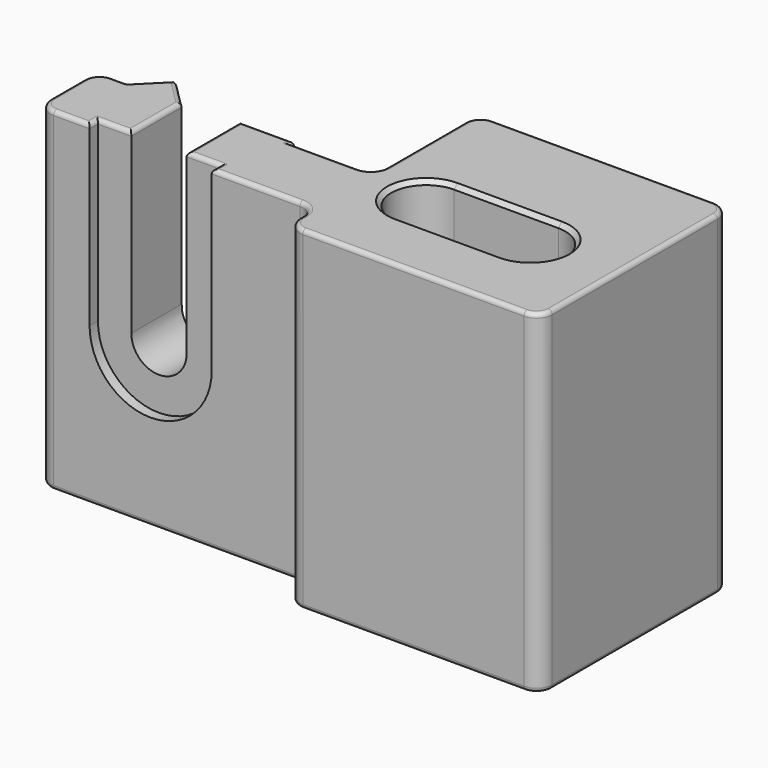
from build123d import *

# Parameters (mm, degrees)
F1_DEPTH      = 32
F2_R          = 0.4
F3_R          = 1.5
F5_DEPTH      = 19.401
F6_DEPTH      = 1
F7_T1_DEPTH   = 1.2843145751
F7_T3_DEPTH   = 4.0870057685
F7_T5_DEPTH   = 4.0870057685
F7_T7_DEPTH   = 8.0359281116
F7_T9_DEPTH   = 4.2
F7_T11_DEPTH  = 2
F7_T13_DEPTH  = 4.45
F7_T15_DEPTH  = 4
F7_T17_DEPTH  = 6.5
F7_T19_DEPTH  = 1.4
F7_T21_DEPTH  = 9.4
F7_T23_DEPTH  = 7.15
F7_T25_DEPTH  = 21.2
F7_T27_DEPTH  = 5.1343145751
F7_T29_DEPTH  = 19.8
F7_T31_DEPTH  = 0.4
F7_T33_DEPTH  = 23.6
F7_T35_DEPTH  = 8.4
F7_T37_DEPTH  = 9.45
F7_T39_DEPTH  = 4.2
F7_T42_ANGLE  = 90
F7_T44_ANGLE  = 90
F7_T46_ANGLE  = 90
F7_T48_ANGLE  = 90
F7_T50_ANGLE  = 90
F7_T52_ANGLE  = 45
F7_T54_ANGLE  = 90
F7_T56_ANGLE  = 90
F7_T58_ANGLE  = 45
F7_T60_ANGLE  = 90
F7_T62_ANGLE  = 90
F7_T64_ANGLE  = 90
F7_T66_ANGLE  = 90
F7_T68_ANGLE  = 90
F7_T70_ANGLE  = 90
F7_T72_ANGLE  = 163.7726416214
F7_T74_ANGLE  = 90
F7_T76_ANGLE  = 90
F7_T78_ANGLE  = 45
F7_T80_ANGLE  = 90
F7_T85_DEPTH  = 5.2
F7_T89_DEPTH  = 3
F7_T96_DEPTH  = 7.5
F7_T100_DEPTH = 2.4
F7_T107_DEPTH = 2.4
F7_T111_DEPTH = 6.1343145751
F7_T118_DEPTH = 7.5
F7_T122_DEPTH = 2.4
F7_T129_DEPTH = 3
F7_T133_DEPTH = 5.2
F10_SIZE      = 0.4
F11_SIZE      = 0.4


# Not quite as in the source:
# - a fillet or chamfer that OpenCascade refuses, or shapes differently, is made with other operations: its cross-section is extruded or revolved along the edge and cut away or added
# - two fillets or chamfers of one size are made in one step


with BuildPart() as f1:
    # F0 (on Top) → F1 (new body)
    with BuildSketch(Plane.XY):
        Polygon((-7.85, 0), (-10.8, 0), (-10.8, -7), (15.8, -7), (15.8, -10.4), (40, -10.4), (40, 12.4), (15.8, 12.4), (15.8, 0), (7.8, 0), (7.8, 0.4), (2.65, 0.4), (2.65, 0), (-2.65, 0), (-4.95, 2.3), (-5.55, 2.3), align=None)
        with BuildLine():
            ThreePointArc((21.6, -4.35), (18.25, -1), (21.6, 2.35))
            Line((21.6, 2.35), (31.6, 2.35))
            ThreePointArc((31.6, 2.35), (34.95, -1), (31.6, -4.35))
            Line((31.6, -4.35), (21.6, -4.35))
        make_face(mode=Mode.SUBTRACT)
    extrude(amount=F1_DEPTH)

    # F2
    f2_edges = [f1.edges().sort_by_distance(p)[0] for p in [
        (-7.85, 0, 16),
        (-2.65, 0, 16),
    ]]
    fillet(f2_edges, radius=F2_R)

    # F3
    f3_edges = [f1.edges().sort_by_distance(p)[0] for p in [
        (-10.8, 0, 16),
        (-10.8, -7, 16),
        (15.8, 12.4, 16),
        (40, 12.4, 16),
        (15.8, -10.4, 16),
        (40, -10.4, 16),
        (15.8, -7, 16),
        (15.8, 0, 16),
    ]]
    fillet(f3_edges, radius=F3_R)

    # F4 (on face) → F5 (cut, through all)
    with BuildSketch(Plane.XZ.offset(7)):
        with BuildLine():
            Line((2.65, 15), (2.65, 32))
            Line((2.65, 32), (-2.65, 32))
            Line((-2.65, 32), (-2.65, 15))
            ThreePointArc((-2.65, 15), (0, 12.35), (2.65, 15))
        make_face()
    extrude(amount=-F5_DEPTH, mode=Mode.SUBTRACT)

    # F4 (on face) → F6 (cut)
    with BuildSketch(Plane.XZ.offset(7)):
        with BuildLine():
            Line((5.85, 32), (2.65, 32))
            Line((2.65, 32), (2.65, 15))
            ThreePointArc((2.65, 15), (0, 12.35), (-2.65, 15))
            Line((-2.65, 15), (-2.65, 32))
            Line((-2.65, 32), (-5.85, 32))
            Line((-5.85, 32), (-5.85, 15))
            ThreePointArc((-5.85, 15), (0, 9.15), (5.85, 15))
            Line((5.85, 15), (5.85, 32))
        make_face()
    extrude(amount=-F6_DEPTH, mode=Mode.SUBTRACT)

    # F7: fillet of radius 0.4 on 55 edges, made by hand

    # F7_s2 → F7_t1 (cut)
    with BuildSketch(Plane.YZ.offset(-9.3)):
        with BuildLine():
            ThreePointArc((0, 31.6), (-0.1171572875, 31.8828427125), (-0.4, 32))
            Line((-0.4, 32), (0, 32))
            Line((0, 32), (0, 31.6))
        make_face()
        with BuildLine():
            ThreePointArc((-0.4, 0), (-0.1171572875, 0.1171572875), (0, 0.4))
            Line((0, 0.4), (0, 0))
            Line((0, 0), (-0.4, 0))
        make_face()
    extrude(amount=F7_T1_DEPTH, mode=Mode.SUBTRACT)

    # F7_s4 → F7_t3 (cut)
    with BuildSketch(Plane(origin=(-0.9178932188, -0.9178932188, 0), x_dir=(0, 0, 1), z_dir=(-0.7071067812, -0.7071067812, 0))):
        with BuildLine():
            ThreePointArc((31.6, 5.5507882323), (31.8828427125, 5.4336309448), (32, 5.1507882323))
            Line((32, 5.1507882323), (32, 5.5507882323))
            Line((32, 5.5507882323), (31.6, 5.5507882323))
        make_face()
        with BuildLine():
            ThreePointArc((0, 5.1507882323), (0.1171572875, 5.4336309448), (0.4, 5.5507882323))
            Line((0.4, 5.5507882323), (0, 5.5507882323))
            Line((0, 5.5507882323), (0, 5.1507882323))
        make_face()
    extrude(amount=F7_T3_DEPTH, mode=Mode.SUBTRACT)

    # F7_s6 → F7_t5 (cut)
    with BuildSketch(Plane(origin=(-1.4421572875, 1.4421572875, 0), x_dir=(0, 0, 1), z_dir=(-0.7071067812, 0.7071067812, 0))):
        with BuildLine():
            ThreePointArc((31.6, -1.8738329701), (31.8828427125, -1.9909902577), (32, -2.2738329701))
            Line((32, -2.2738329701), (32, -1.8738329701))
            Line((32, -1.8738329701), (31.6, -1.8738329701))
        make_face()
        with BuildLine():
            ThreePointArc((0, -2.2738329701), (0.1171572875, -1.9909902577), (0.4, -1.8738329701))
            Line((0.4, -1.8738329701), (0, -1.8738329701))
            Line((0, -1.8738329701), (0, -2.2738329701))
        make_face()
    extrude(amount=F7_T5_DEPTH, mode=Mode.SUBTRACT)

    # F7_s8 → F7_t7 (cut)
    with BuildSketch(Plane.XZ.offset(-1.0359281116)):
        with BuildLine():
            ThreePointArc((-2.65, 31.6), (-2.7671572875, 31.8828427125), (-3.05, 32))
            Line((-3.05, 32), (-2.65, 32))
            Line((-2.65, 32), (-2.65, 31.6))
        make_face()
    extrude(amount=F7_T7_DEPTH, mode=Mode.SUBTRACT)

    # F7_s10 → F7_t9 (cut)
    with BuildSketch(Plane.YZ.offset(-5.85)):
        with BuildLine():
            ThreePointArc((-6, 31.6), (-5.8828427125, 31.8828427125), (-5.6, 32))
            Line((-5.6, 32), (-6, 32))
            Line((-6, 32), (-6, 31.6))
        make_face()
    extrude(amount=F7_T9_DEPTH, mode=Mode.SUBTRACT)

    # F7_s12 → F7_t11 (cut)
    with BuildSketch(Plane.XZ.offset(6)):
        with BuildLine():
            ThreePointArc((-6.25, 32), (-5.9671572875, 31.8828427125), (-5.85, 31.6))
            Line((-5.85, 31.6), (-5.85, 32))
            Line((-5.85, 32), (-6.25, 32))
        make_face()
        with BuildLine():
            ThreePointArc((6.25, 32), (5.9671572875, 31.8828427125), (5.85, 31.6))
            Line((5.85, 31.6), (5.85, 32))
            Line((5.85, 32), (6.25, 32))
        make_face()
    extrude(amount=F7_T11_DEPTH, mode=Mode.SUBTRACT)

    # F7_s14 → F7_t13 (cut)
    with BuildSketch(Plane.YZ.offset(-9.3)):
        with BuildLine():
            ThreePointArc((-7, 31.6), (-6.8828427125, 31.8828427125), (-6.6, 32))
            Line((-6.6, 32), (-7, 32))
            Line((-7, 32), (-7, 31.6))
        make_face()
    extrude(amount=F7_T13_DEPTH, mode=Mode.SUBTRACT)

    # F7_s16 → F7_t15 (cut)
    with BuildSketch(Plane.XZ.offset(1.5)):
        with BuildLine():
            ThreePointArc((-10.8, 31.6), (-10.6828427125, 31.8828427125), (-10.4, 32))
            Line((-10.4, 32), (-10.8, 32))
            Line((-10.8, 32), (-10.8, 31.6))
        make_face()
        with BuildLine():
            ThreePointArc((-10.4, 0), (-10.6828427125, 0.1171572875), (-10.8, 0.4))
            Line((-10.8, 0.4), (-10.8, 0))
            Line((-10.8, 0), (-10.4, 0))
        make_face()
    extrude(amount=F7_T15_DEPTH, mode=Mode.SUBTRACT)

    # F7_s18 → F7_t17 (cut)
    with BuildSketch(Plane.YZ.offset(7.8)):
        with BuildLine():
            ThreePointArc((-0.4, 0), (-0.1171572875, 0.1171572875), (0, 0.4))
            Line((0, 0.4), (0, 0))
            Line((0, 0), (-0.4, 0))
        make_face()
        with BuildLine():
            ThreePointArc((0, 31.6), (-0.1171572875, 31.8828427125), (-0.4, 32))
            Line((-0.4, 32), (0, 32))
            Line((0, 32), (0, 31.6))
        make_face()
    extrude(amount=F7_T17_DEPTH, mode=Mode.SUBTRACT)

    # F7_s20 → F7_t19 (cut)
    with BuildSketch(Plane.XZ.offset(-1.4)):
        with BuildLine():
            ThreePointArc((7.4, 0), (7.6828427125, 0.1171572875), (7.8, 0.4))
            Line((7.8, 0.4), (7.8, 0))
            Line((7.8, 0), (7.4, 0))
        make_face()
        with BuildLine():
            ThreePointArc((3.05, 0), (2.7671572875, 0.1171572875), (2.65, 0.4))
            Line((2.65, 0.4), (2.65, 0))
            Line((2.65, 0), (3.05, 0))
        make_face()
        with BuildLine():
            ThreePointArc((7.8, 31.6), (7.6828427125, 31.8828427125), (7.4, 32))
            Line((7.4, 32), (7.8, 32))
            Line((7.8, 32), (7.8, 31.6))
        make_face()
    extrude(amount=F7_T19_DEPTH, mode=Mode.SUBTRACT)

    # F7_s22 → F7_t21 (cut)
    with BuildSketch(Plane.XZ.offset(-10.9)):
        with BuildLine():
            ThreePointArc((16.2, 0), (15.9171572875, 0.1171572875), (15.8, 0.4))
            Line((15.8, 0.4), (15.8, 0))
            Line((15.8, 0), (16.2, 0))
        make_face()
        with BuildLine():
            ThreePointArc((15.8, 31.6), (15.9171572875, 31.8828427125), (16.2, 32))
            Line((16.2, 32), (15.8, 32))
            Line((15.8, 32), (15.8, 31.6))
        make_face()
    extrude(amount=F7_T21_DEPTH, mode=Mode.SUBTRACT)

    # F7_s24 → F7_t23 (cut)
    with BuildSketch(Plane.YZ.offset(1.65)):
        with BuildLine():
            ThreePointArc((0, 0), (0.2828427125, 0.1171572875), (0.4, 0.4))
            Line((0.4, 0.4), (0.4, 0))
            Line((0.4, 0), (0, 0))
        make_face()
        with BuildLine():
            ThreePointArc((0.4, 31.6), (0.2828427125, 31.8828427125), (0, 32))
            Line((0, 32), (0.4, 32))
            Line((0.4, 32), (0.4, 31.6))
        make_face()
    extrude(amount=F7_T23_DEPTH, mode=Mode.SUBTRACT)

    # F7_s26 → F7_t25 (cut)
    with BuildSketch(Plane.YZ.offset(17.3)):
        with BuildLine():
            ThreePointArc((12, 0), (12.2828427125, 0.1171572875), (12.4, 0.4))
            Line((12.4, 0.4), (12.4, 0))
            Line((12.4, 0), (12, 0))
        make_face()
        with BuildLine():
            ThreePointArc((-10, 0), (-10.2828427125, 0.1171572875), (-10.4, 0.4))
            Line((-10.4, 0.4), (-10.4, 0))
            Line((-10.4, 0), (-10, 0))
        make_face()
        with BuildLine():
            ThreePointArc((12.4, 31.6), (12.2828427125, 31.8828427125), (12, 32))
            Line((12, 32), (12.4, 32))
            Line((12.4, 32), (12.4, 31.6))
        make_face()
        with BuildLine():
            ThreePointArc((-10.4, 31.6), (-10.2828427125, 31.8828427125), (-10, 32))
            Line((-10, 32), (-10.4, 32))
            Line((-10.4, 32), (-10.4, 31.6))
        make_face()
    extrude(amount=F7_T25_DEPTH, mode=Mode.SUBTRACT)

    # F7_s28 → F7_t27 (cut)
    with BuildSketch(Plane.YZ.offset(-2.4843145751)):
        with BuildLine():
            ThreePointArc((-0.4, 0), (-0.1171572875, 0.1171572875), (0, 0.4))
            Line((0, 0.4), (0, 0))
            Line((0, 0), (-0.4, 0))
        make_face()
    extrude(amount=F7_T27_DEPTH, mode=Mode.SUBTRACT)

    # F7_s30 → F7_t29 (cut)
    with BuildSketch(Plane.XZ.offset(-10.9)):
        with BuildLine():
            ThreePointArc((39.6, 0), (39.8828427125, 0.1171572875), (40, 0.4))
            Line((40, 0.4), (40, 0))
            Line((40, 0), (39.6, 0))
        make_face()
        with BuildLine():
            ThreePointArc((40, 31.6), (39.8828427125, 31.8828427125), (39.6, 32))
            Line((39.6, 32), (40, 32))
            Line((40, 32), (40, 31.6))
        make_face()
    extrude(amount=F7_T29_DEPTH, mode=Mode.SUBTRACT)

    # F7_s32 → F7_t31 (cut)
    with BuildSketch(Plane.XZ.offset(8.5)):
        with BuildLine():
            ThreePointArc((16.2, 0), (15.9171572875, 0.1171572875), (15.8, 0.4))
            Line((15.8, 0.4), (15.8, 0))
            Line((15.8, 0), (16.2, 0))
        make_face()
        with BuildLine():
            ThreePointArc((15.8, 31.6), (15.9171572875, 31.8828427125), (16.2, 32))
            Line((16.2, 32), (15.8, 32))
            Line((15.8, 32), (15.8, 31.6))
        make_face()
    extrude(amount=F7_T31_DEPTH, mode=Mode.SUBTRACT)

    # F7_s34 → F7_t33 (cut)
    with BuildSketch(Plane.YZ.offset(-9.3)):
        with BuildLine():
            ThreePointArc((-6.6, 0), (-6.8828427125, 0.1171572875), (-7, 0.4))
            Line((-7, 0.4), (-7, 0))
            Line((-7, 0), (-6.6, 0))
        make_face()
    extrude(amount=F7_T33_DEPTH, mode=Mode.SUBTRACT)

    # F7_s36 → F7_t35 (cut)
    with BuildSketch(Plane.XZ.offset(-1.4)):
        with BuildLine():
            ThreePointArc((2.65, 31.6), (2.7671572875, 31.8828427125), (3.05, 32))
            Line((3.05, 32), (2.65, 32))
            Line((2.65, 32), (2.65, 31.6))
        make_face()
    extrude(amount=F7_T35_DEPTH, mode=Mode.SUBTRACT)

    # F7_s38 → F7_t37 (cut)
    with BuildSketch(Plane.YZ.offset(4.85)):
        with BuildLine():
            ThreePointArc((-7, 31.6), (-6.8828427125, 31.8828427125), (-6.6, 32))
            Line((-6.6, 32), (-7, 32))
            Line((-7, 32), (-7, 31.6))
        make_face()
    extrude(amount=F7_T37_DEPTH, mode=Mode.SUBTRACT)

    # F7_s40 → F7_t39 (cut)
    with BuildSketch(Plane.YZ.offset(1.65)):
        with BuildLine():
            ThreePointArc((-5.6, 32), (-5.8828427125, 31.8828427125), (-6, 31.6))
            Line((-6, 31.6), (-6, 32))
            Line((-6, 32), (-5.6, 32))
        make_face()
    extrude(amount=F7_T39_DEPTH, mode=Mode.SUBTRACT)

    # F7_s41 → F7_t42 (revolve, cut)
    with BuildSketch(Plane.YZ.offset(-9.3)):
        with BuildLine():
            ThreePointArc((0, 31.6), (-0.1171572875, 31.8828427125), (-0.4, 32))
            Line((-0.4, 32), (0, 32))
            Line((0, 32), (0, 31.6))
        make_face()
    revolve(axis=Axis((-9.3, -1.5, 32), (0, 0, 1)), revolution_arc=F7_T42_ANGLE, mode=Mode.SUBTRACT)

    # F7_s43 → F7_t44 (revolve, cut)
    with BuildSketch(Plane.XZ.offset(5.5)):
        with BuildLine():
            ThreePointArc((-10.8, 31.6), (-10.6828427125, 31.8828427125), (-10.4, 32))
            Line((-10.4, 32), (-10.8, 32))
            Line((-10.8, 32), (-10.8, 31.6))
        make_face()
    revolve(axis=Axis((-9.3, -5.5, 32), (0, 0, 1)), revolution_arc=F7_T44_ANGLE, mode=Mode.SUBTRACT)

    # F7_s45 → F7_t46 (revolve, cut)
    with BuildSketch(Plane.YZ.offset(14.3)):
        with BuildLine():
            ThreePointArc((-0.4, 0), (-0.1171572875, 0.1171572875), (0, 0.4))
            Line((0, 0.4), (0, 0))
            Line((0, 0), (-0.4, 0))
        make_face()
    revolve(axis=Axis((14.3, 1.5, 0), (0, 0, 1)), revolution_arc=F7_T46_ANGLE, mode=Mode.SUBTRACT)

    # F7_s47 → F7_t48 (revolve, cut)
    with BuildSketch(Plane.XZ.offset(-10.9)):
        with BuildLine():
            ThreePointArc((16.2, 0), (15.9171572875, 0.1171572875), (15.8, 0.4))
            Line((15.8, 0.4), (15.8, 0))
            Line((15.8, 0), (16.2, 0))
        make_face()
    revolve(axis=Axis((17.3, 10.9, 0), (0, 0, -1)), revolution_arc=F7_T48_ANGLE, mode=Mode.SUBTRACT)

    # F7_s49 → F7_t50 (revolve, cut)
    with BuildSketch(Plane.YZ.offset(38.5)):
        with BuildLine():
            ThreePointArc((12, 0), (12.2828427125, 0.1171572875), (12.4, 0.4))
            Line((12.4, 0.4), (12.4, 0))
            Line((12.4, 0), (12, 0))
        make_face()
    revolve(axis=Axis((38.5, 10.9, 0), (0, 0, -1)), revolution_arc=F7_T50_ANGLE, mode=Mode.SUBTRACT)

    # F7_s51 → F7_t52 (revolve, cut)
    with BuildSketch(Plane.YZ.offset(-2.4843145751)):
        with BuildLine():
            ThreePointArc((-0.4, 0), (-0.1171572875, 0.1171572875), (0, 0.4))
            Line((0, 0.4), (0, 0))
            Line((0, 0), (-0.4, 0))
        make_face()
    revolve(axis=Axis((-2.4843145751, 0.4, 0), (0, 0, -1)), revolution_arc=F7_T52_ANGLE, mode=Mode.SUBTRACT)

    # F7_s53 → F7_t54 (revolve, cut)
    with BuildSketch(Plane.XZ.offset(8.9)):
        with BuildLine():
            ThreePointArc((39.6, 0), (39.8828427125, 0.1171572875), (40, 0.4))
            Line((40, 0.4), (40, 0))
            Line((40, 0), (39.6, 0))
        make_face()
    revolve(axis=Axis((38.5, -8.9, 0), (0, 0, -1)), revolution_arc=F7_T54_ANGLE, mode=Mode.SUBTRACT)

    # F7_s55 → F7_t56 (revolve, cut)
    with BuildSketch(Plane.YZ.offset(17.3)):
        with BuildLine():
            ThreePointArc((-10, 0), (-10.2828427125, 0.1171572875), (-10.4, 0.4))
            Line((-10.4, 0.4), (-10.4, 0))
            Line((-10.4, 0), (-10, 0))
        make_face()
    revolve(axis=Axis((17.3, -8.9, 0), (0, 0, -1)), revolution_arc=F7_T56_ANGLE, mode=Mode.SUBTRACT)

    # F7_s57 → F7_t58 (revolve, cut)
    with BuildSketch(Plane(origin=(-3.8078427125, -3.8078427125, 0), x_dir=(0, 0, 1), z_dir=(0.7071067812, 0.7071067812, 0))):
        with BuildLine():
            ThreePointArc((0, -5.1507882323), (0.1171572875, -5.4336309448), (0.4, -5.5507882323))
            Line((0.4, -5.5507882323), (0, -5.5507882323))
            Line((0, -5.5507882323), (0, -5.1507882323))
        make_face()
    revolve(axis=Axis((-8.0156854249, 0.4, 0), (0, 0, -1)), revolution_arc=F7_T58_ANGLE, mode=Mode.SUBTRACT)

    # F7_s59 → F7_t60 (revolve, cut)
    with BuildSketch(Plane.YZ.offset(14.3)):
        with BuildLine():
            ThreePointArc((-6.6, 0), (-6.8828427125, 0.1171572875), (-7, 0.4))
            Line((-7, 0.4), (-7, 0))
            Line((-7, 0), (-6.6, 0))
        make_face()
    revolve(axis=Axis((14.3, -8.5, 0), (0, 0, -1)), revolution_arc=F7_T60_ANGLE, mode=Mode.SUBTRACT)

    # F7_s61 → F7_t62 (revolve, cut)
    with BuildSketch(Plane.YZ.offset(-9.3)):
        with BuildLine():
            ThreePointArc((-0.4, 0), (-0.1171572875, 0.1171572875), (0, 0.4))
            Line((0, 0.4), (0, 0))
            Line((0, 0), (-0.4, 0))
        make_face()
    revolve(axis=Axis((-9.3, -1.5, 0), (0, 0, 1)), revolution_arc=F7_T62_ANGLE, mode=Mode.SUBTRACT)

    # F7_s63 → F7_t64 (revolve, cut)
    with BuildSketch(Plane.XZ.offset(5.5)):
        with BuildLine():
            ThreePointArc((-10.4, 0), (-10.6828427125, 0.1171572875), (-10.8, 0.4))
            Line((-10.8, 0.4), (-10.8, 0))
            Line((-10.8, 0), (-10.4, 0))
        make_face()
    revolve(axis=Axis((-9.3, -5.5, 0), (0, 0, 1)), revolution_arc=F7_T64_ANGLE, mode=Mode.SUBTRACT)

    # F7_s65 → F7_t66 (revolve, cut)
    with BuildSketch(Plane.YZ.offset(14.3)):
        with BuildLine():
            ThreePointArc((0, 31.6), (-0.1171572875, 31.8828427125), (-0.4, 32))
            Line((-0.4, 32), (0, 32))
            Line((0, 32), (0, 31.6))
        make_face()
    revolve(axis=Axis((14.3, 1.5, 32), (0, 0, 1)), revolution_arc=F7_T66_ANGLE, mode=Mode.SUBTRACT)

    # F7_s67 → F7_t68 (revolve, cut)
    with BuildSketch(Plane.XZ.offset(-10.9)):
        with BuildLine():
            ThreePointArc((15.8, 31.6), (15.9171572875, 31.8828427125), (16.2, 32))
            Line((16.2, 32), (15.8, 32))
            Line((15.8, 32), (15.8, 31.6))
        make_face()
    revolve(axis=Axis((17.3, 10.9, 32), (0, 0, -1)), revolution_arc=F7_T68_ANGLE, mode=Mode.SUBTRACT)

    # F7_s69 → F7_t70 (revolve, cut)
    with BuildSketch(Plane.YZ.offset(38.5)):
        with BuildLine():
            ThreePointArc((12.4, 31.6), (12.2828427125, 31.8828427125), (12, 32))
            Line((12, 32), (12.4, 32))
            Line((12.4, 32), (12.4, 31.6))
        make_face()
    revolve(axis=Axis((38.5, 10.9, 32), (0, 0, -1)), revolution_arc=F7_T70_ANGLE, mode=Mode.SUBTRACT)

    # F7_s71 → F7_t72 (revolve, cut)
    with BuildSketch(Plane(origin=(-0.7443380199, 1.3554785605, 0), x_dir=(0, 0, 1), z_dir=(-0.4813351882, 0.8765366145, 0))):
        with BuildLine():
            ThreePointArc((31.6, -1.5850586117), (31.8828427125, -1.4679013242), (32, -1.1850586117))
            Line((32, -1.1850586117), (32, -1.5850586117))
            Line((32, -1.5850586117), (31.6, -1.5850586117))
        make_face()
    revolve(axis=Axis((-2.4843145751, 0.4, 32), (0, 0, -1)), revolution_arc=F7_T72_ANGLE, mode=Mode.SUBTRACT)

    # F7_s73 → F7_t74 (revolve, cut)
    with BuildSketch(Plane.XZ.offset(8.9)):
        with BuildLine():
            ThreePointArc((40, 31.6), (39.8828427125, 31.8828427125), (39.6, 32))
            Line((39.6, 32), (40, 32))
            Line((40, 32), (40, 31.6))
        make_face()
    revolve(axis=Axis((38.5, -8.9, 32), (0, 0, -1)), revolution_arc=F7_T74_ANGLE, mode=Mode.SUBTRACT)

    # F7_s75 → F7_t76 (revolve, cut)
    with BuildSketch(Plane.YZ.offset(17.3)):
        with BuildLine():
            ThreePointArc((-10.4, 31.6), (-10.2828427125, 31.8828427125), (-10, 32))
            Line((-10, 32), (-10.4, 32))
            Line((-10.4, 32), (-10.4, 31.6))
        make_face()
    revolve(axis=Axis((17.3, -8.9, 32), (0, 0, -1)), revolution_arc=F7_T76_ANGLE, mode=Mode.SUBTRACT)

    # F7_s77 → F7_t78 (revolve, cut)
    with BuildSketch(Plane(origin=(-3.8078427125, -3.8078427125, 0), x_dir=(0, 0, 1), z_dir=(0.7071067812, 0.7071067812, 0))):
        with BuildLine():
            ThreePointArc((31.6, -5.5507882323), (31.8828427125, -5.4336309448), (32, -5.1507882323))
            Line((32, -5.1507882323), (32, -5.5507882323))
            Line((32, -5.5507882323), (31.6, -5.5507882323))
        make_face()
    revolve(axis=Axis((-8.0156854249, 0.4, 32), (0, 0, -1)), revolution_arc=F7_T78_ANGLE, mode=Mode.SUBTRACT)

    # F7_s79 → F7_t80 (revolve, cut)
    with BuildSketch(Plane.YZ.offset(14.3)):
        with BuildLine():
            ThreePointArc((-7, 31.6), (-6.8828427125, 31.8828427125), (-6.6, 32))
            Line((-6.6, 32), (-7, 32))
            Line((-7, 32), (-7, 31.6))
        make_face()
    revolve(axis=Axis((14.3, -8.5, 32), (0, 0, -1)), revolution_arc=F7_T80_ANGLE, mode=Mode.SUBTRACT)


with BuildPart() as f7_tool83:
    # F7_s84 → F7_t85 (new body)
    with BuildSketch(Plane.YZ.offset(-1.65)):
        with BuildLine():
            ThreePointArc((-6, 31.6), (-5.8828427125, 31.8828427125), (-5.6, 32))
            Line((-5.6, 32), (-6, 32))
            Line((-6, 32), (-6, 31.6))
        make_face()
    extrude(amount=-F7_T85_DEPTH)

    split(bisect_by=Plane.YZ.offset(-5.85), keep=Keep.BOTTOM)


with BuildPart() as f7_tool87:
    # F7_s88 → F7_t89 (new body)
    with BuildSketch(Plane.XZ.offset(8)):
        with BuildLine():
            ThreePointArc((-6.25, 32), (-5.9671572875, 31.8828427125), (-5.85, 31.6))
            Line((-5.85, 31.6), (-5.85, 32))
            Line((-5.85, 32), (-6.25, 32))
        make_face()
    extrude(amount=-F7_T89_DEPTH)

    split(bisect_by=Plane.XZ.offset(6), keep=Keep.BOTTOM)


with BuildPart() as f7_tool83_1:
    add(f7_tool83.part)

    # F7_t91: intersect F7_tool87
    add(f7_tool87.part, mode=Mode.INTERSECT)


with BuildPart() as f1_1:
    add(f1.part)

    # F7_t81: cut F7_tool83
    add(f7_tool83_1.part, mode=Mode.SUBTRACT)


with BuildPart() as f7_tool94:
    # F7_s95 → F7_t96 (new body)
    with BuildSketch(Plane.YZ.offset(14.3)):
        with BuildLine():
            ThreePointArc((-0.4, 0), (-0.1171572875, 0.1171572875), (0, 0.4))
            Line((0, 0.4), (0, 0))
            Line((0, 0), (-0.4, 0))
        make_face()
    extrude(amount=-F7_T96_DEPTH)

    split(bisect_by=Plane.YZ.offset(7.8), keep=Keep.BOTTOM)


with BuildPart() as f7_tool98:
    # F7_s99 → F7_t100 (new body)
    with BuildSketch(Plane.XZ.offset(1)):
        with BuildLine():
            ThreePointArc((7.4, 0), (7.6828427125, 0.1171572875), (7.8, 0.4))
            Line((7.8, 0.4), (7.8, 0))
            Line((7.8, 0), (7.4, 0))
        make_face()
    extrude(amount=-F7_T100_DEPTH)

    split(bisect_by=Plane.XZ, keep=Keep.TOP)


with BuildPart() as f7_tool94_1:
    add(f7_tool94.part)

    # F7_t102: intersect F7_tool98
    add(f7_tool98.part, mode=Mode.INTERSECT)


with BuildPart() as f1_2:
    add(f1_1.part)

    # F7_t92: cut F7_tool94
    add(f7_tool94_1.part, mode=Mode.SUBTRACT)


with BuildPart() as f7_tool105:
    # F7_s106 → F7_t107 (new body)
    with BuildSketch(Plane.XZ.offset(-1.4)):
        with BuildLine():
            ThreePointArc((3.05, 0), (2.7671572875, 0.1171572875), (2.65, 0.4))
            Line((2.65, 0.4), (2.65, 0))
            Line((2.65, 0), (3.05, 0))
        make_face()
    extrude(amount=F7_T107_DEPTH)

    split(bisect_by=Plane.XZ, keep=Keep.TOP)


with BuildPart() as f7_tool109:
    # F7_s110 → F7_t111 (new body)
    with BuildSketch(Plane.YZ.offset(3.65)):
        with BuildLine():
            ThreePointArc((-0.4, 0), (-0.1171572875, 0.1171572875), (0, 0.4))
            Line((0, 0.4), (0, 0))
            Line((0, 0), (-0.4, 0))
        make_face()
    extrude(amount=-F7_T111_DEPTH)

    split(bisect_by=Plane.YZ.offset(2.65), keep=Keep.TOP)


with BuildPart() as f7_tool105_1:
    add(f7_tool105.part)

    # F7_t113: intersect F7_tool109
    add(f7_tool109.part, mode=Mode.INTERSECT)


with BuildPart() as f1_3:
    add(f1_2.part)

    # F7_t103: cut F7_tool105
    add(f7_tool105_1.part, mode=Mode.SUBTRACT)


with BuildPart() as f7_tool116:
    # F7_s117 → F7_t118 (new body)
    with BuildSketch(Plane.YZ.offset(14.3)):
        with BuildLine():
            ThreePointArc((0, 31.6), (-0.1171572875, 31.8828427125), (-0.4, 32))
            Line((-0.4, 32), (0, 32))
            Line((0, 32), (0, 31.6))
        make_face()
    extrude(amount=-F7_T118_DEPTH)

    split(bisect_by=Plane.YZ.offset(7.8), keep=Keep.BOTTOM)


with BuildPart() as f7_tool120:
    # F7_s121 → F7_t122 (new body)
    with BuildSketch(Plane.XZ.offset(1)):
        with BuildLine():
            ThreePointArc((7.8, 31.6), (7.6828427125, 31.8828427125), (7.4, 32))
            Line((7.4, 32), (7.8, 32))
            Line((7.8, 32), (7.8, 31.6))
        make_face()
    extrude(amount=-F7_T122_DEPTH)

    split(bisect_by=Plane.XZ, keep=Keep.TOP)


with BuildPart() as f7_tool116_1:
    add(f7_tool116.part)

    # F7_t124: intersect F7_tool120
    add(f7_tool120.part, mode=Mode.INTERSECT)


with BuildPart() as f1_4:
    add(f1_3.part)

    # F7_t114: cut F7_tool116
    add(f7_tool116_1.part, mode=Mode.SUBTRACT)


with BuildPart() as f7_tool127:
    # F7_s128 → F7_t129 (new body)
    with BuildSketch(Plane.XZ.offset(8)):
        with BuildLine():
            ThreePointArc((6.25, 32), (5.9671572875, 31.8828427125), (5.85, 31.6))
            Line((5.85, 31.6), (5.85, 32))
            Line((5.85, 32), (6.25, 32))
        make_face()
    extrude(amount=-F7_T129_DEPTH)

    split(bisect_by=Plane.XZ.offset(6), keep=Keep.BOTTOM)


with BuildPart() as f7_tool131:
    # F7_s132 → F7_t133 (new body)
    with BuildSketch(Plane.YZ.offset(6.85)):
        with BuildLine():
            ThreePointArc((-5.6, 32), (-5.8828427125, 31.8828427125), (-6, 31.6))
            Line((-6, 31.6), (-6, 32))
            Line((-6, 32), (-5.6, 32))
        make_face()
    extrude(amount=-F7_T133_DEPTH)

    split(bisect_by=Plane.YZ.offset(5.85), keep=Keep.TOP)


with BuildPart() as f7_tool127_1:
    add(f7_tool127.part)

    # F7_t135: intersect F7_tool131
    add(f7_tool131.part, mode=Mode.INTERSECT)


with BuildPart() as f1_5:
    add(f1_4.part)

    # F7_t125: cut F7_tool127
    add(f7_tool127_1.part, mode=Mode.SUBTRACT)

    # F10
    f10_edges = [f1_5.edges().sort_by_distance(p)[0] for p in [
        (18.25, -1, 0),
    ]]
    chamfer(f10_edges, length=F10_SIZE)

    # F11
    f11_edges = [f1_5.edges().sort_by_distance(p)[0] for p in [
        (18.25, -1, 32),
        (26.6, -4.35, 32),
        (26.6, 2.35, 32),
        (34.95, -1, 32),
    ]]
    chamfer(f11_edges, length=F11_SIZE)


solid = f1_5.part
